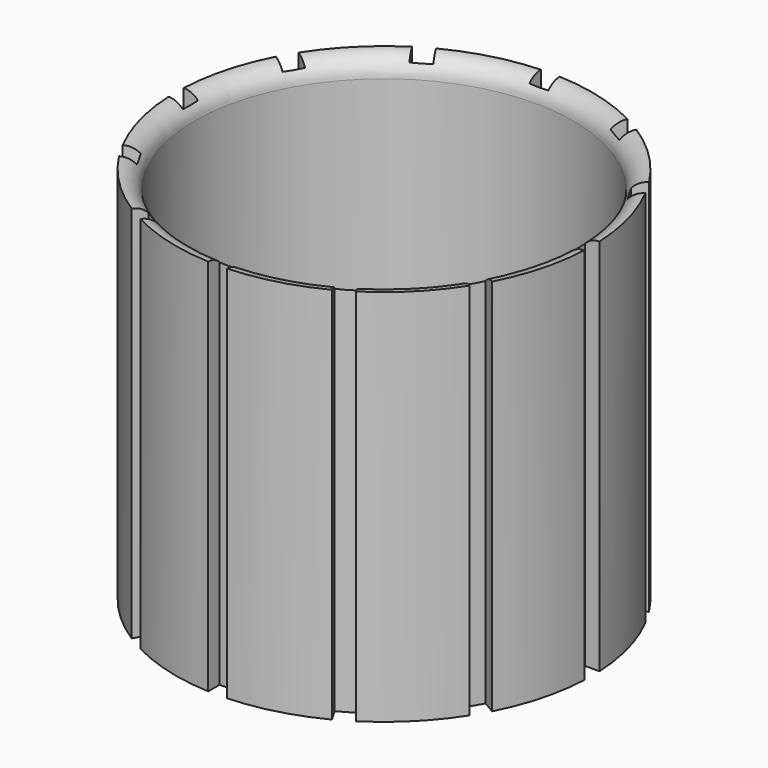
from build123d import *

# Parameters (mm, degrees)
F0_R            = 55
F0_R_2          = 50
F1_DEPTH        = 100
F2_R            = 50
F3_DEPTH        = 1.2
F4_W            = 5
F4_H            = 5
F5_DEPTH        = 200.6
F5_COPIES_COUNT = 12


# Not quite as in the source:
# - a fillet or chamfer that OpenCascade refuses, or shapes differently, is made with other operations: its cross-section is extruded or revolved along the edge and cut away or added
# - a pattern or mirror of a feature is missing from the dataset's text; its kind, count and spacing are read off the source's solid


with BuildPart() as f1:
    # F0 (on Top) → F1 (new body)
    with BuildSketch(Plane.XY):
        Circle(F0_R)
        Circle(F0_R_2, mode=Mode.SUBTRACT)
    extrude(amount=F1_DEPTH)

    # F2 (on Top) → F3 (join)
    with BuildSketch(Plane.XY):
        Circle(F2_R)
    extrude(amount=F3_DEPTH)

    # F4 (on Top) → F5 (cut)
    with BuildSketch(Plane.XY):
        with Locations((0, 53.6743810624)):
            Rectangle(F4_W, F4_H)
    f5 = extrude(amount=F5_DEPTH, mode=Mode.SUBTRACT)

    # F5_copies: F5 ×12 about axis
    f5_copies_axis = Axis((0, 0, 0), (0, 0, 1))
    for i in range(1, F5_COPIES_COUNT):
        add(f5.rotate(f5_copies_axis, i * 360 / F5_COPIES_COUNT), mode=Mode.SUBTRACT)

    # F7: fillet of radius 5 on 1 edges, made by hand

    # F7_s1 → F7_t2 (revolve, cut)
    with BuildSketch(Plane.XZ):
        with BuildLine():
            ThreePointArc((55, 100), (51.4644660941, 98.5355339059), (50, 95))
            Line((50, 95), (50, 100))
            Line((50, 100), (55, 100))
        make_face()
    revolve(axis=Axis((0, 0, 100), (0, 0, 1)), mode=Mode.SUBTRACT)


solid = f1.part
